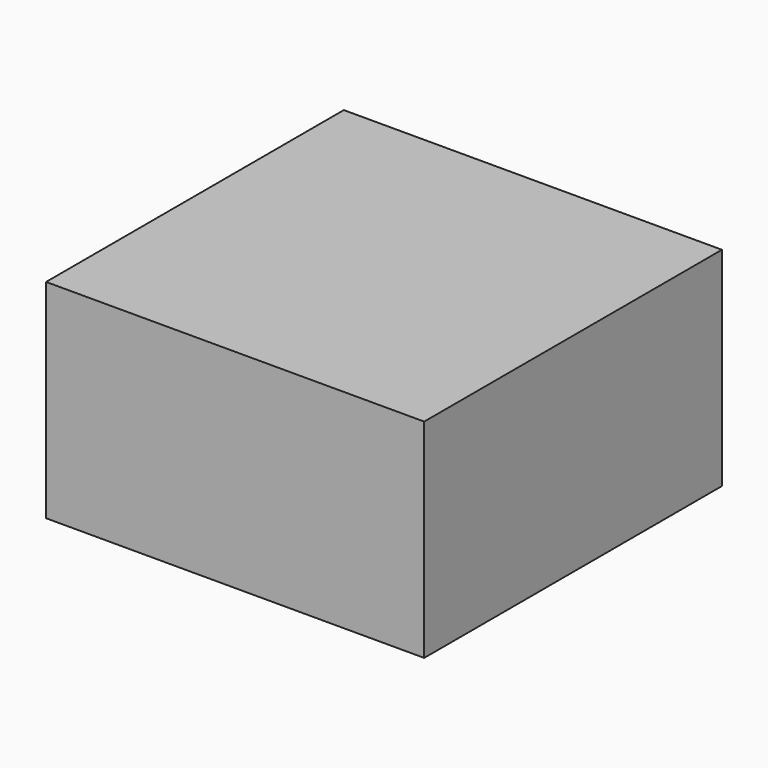
from build123d import *

# Parameters (mm, degrees)
F0_W     = 69.8630958796
F0_H     = 137.5265717506
F2_DEPTH = 76.8858


# Not quite as in the source:
# - the program builds the solid bodies; features that only make, move or delete a surface that nothing else refers to are left out


with BuildPart() as f2:
    # F0 (on Top) → F2 (new body)
    with BuildSketch(Plane.XY):
        with Locations((34.9315479398, 0)):
            Rectangle(F0_W, F0_H)
        with Locations((-34.9315479398, 0)):
            Rectangle(F0_W, F0_H)
    extrude(amount=-F2_DEPTH)


solid = f2.part
